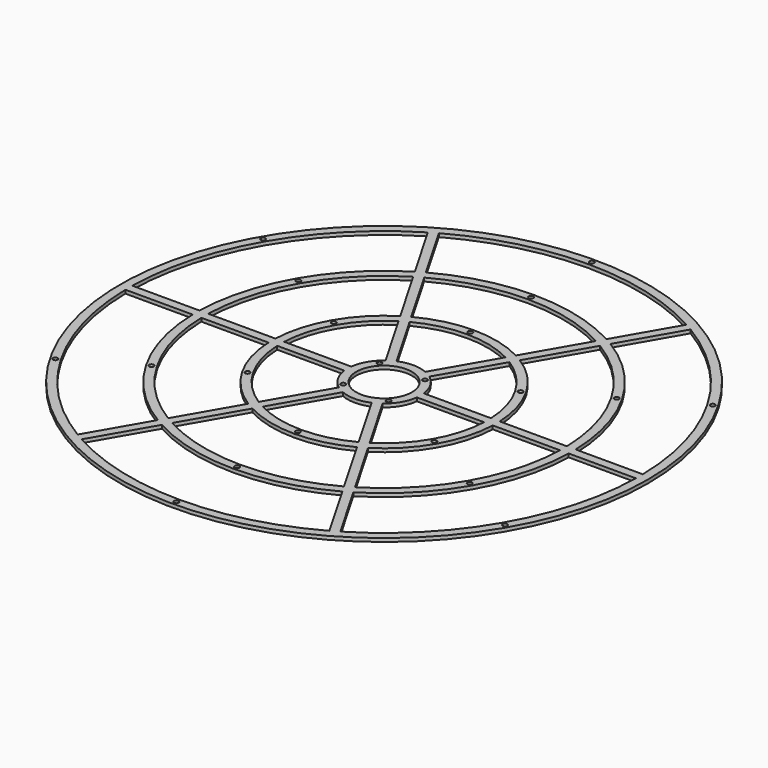
from build123d import *

# Parameters (mm, degrees)
F0_R            = 241.3
F0_R_2          = 25.4
F1_DEPTH        = 3.175
F2_R            = 2.15265
F3_DEPTH        = 3.175
F3_COPIES_COUNT = 6
F4_R            = 2.15265
F5_DEPTH        = 3.175


# Not quite as in the source:
# - a pattern or mirror of a feature is missing from the dataset's text; its kind, count and spacing are read off the source's solid


with BuildPart() as f1:
    # F0 (on Top) → F1 (new body)
    with BuildSketch(Plane.XY):
        Circle(F0_R)
        Circle(F0_R_2, mode=Mode.SUBTRACT)
    extrude(amount=F1_DEPTH)

    # F2 (on face) → F3 (cut, through all)
    with BuildSketch(Plane.XY.offset(3.175)):
        with BuildLine():
            ThreePointArc((13.1131726267, -30.6501812378), (0, -33.3375), (-13.1131726267, -30.6501812378))
            Line((-13.1131726267, -30.6501812378), (-43.8387272582, -83.8684029504))
            ThreePointArc((-43.8387272582, -83.8684029504), (0, -94.6347875841), (43.8387272582, -83.8684029504))
            Line((43.8387272582, -83.8684029504), (13.1131726267, -30.6501812378))
        make_face()
        with BuildLine():
            Line((-82.5017818898, -150.8347779481), (-113.2273365214, -204.0529996607))
            ThreePointArc((-113.2273365214, -204.0529996607), (0, -233.3625), (113.2273365214, -204.0529996607))
            Line((113.2273365214, -204.0529996607), (82.5017818898, -150.8347779481))
            ThreePointArc((82.5017818898, -150.8347779481), (0, -171.923454635), (-82.5017818898, -150.8347779481))
        make_face()
        with BuildLine():
            ThreePointArc((47.8074772582, -90.742479593), (0, -102.5658446291), (-47.8074772582, -90.742479593))
            Line((-47.8074772582, -90.742479593), (-78.5330318898, -143.9607013056))
            ThreePointArc((-78.5330318898, -143.9607013056), (0, -163.9881721899), (78.5330318898, -143.9607013056))
            Line((78.5330318898, -143.9607013056), (47.8074772582, -90.742479593))
        make_face()
        with Locations((0, -98.6003161066)):
            Circle(F2_R)
        with Locations((0, -167.9558134125)):
            Circle(F2_R)
        with Locations((0, -237.33125)):
            Circle(F2_R)
    f3 = extrude(amount=-F3_DEPTH, mode=Mode.SUBTRACT)

    # F3_copies: F3 ×6 about axis
    f3_copies_axis = Axis((0, 0, 0), (0, 0, 1))
    for i in range(1, F3_COPIES_COUNT):
        add(f3.rotate(f3_copies_axis, i * 360 / F3_COPIES_COUNT), mode=Mode.SUBTRACT)

    # F4 (on face) → F5 (cut, through all)
    with BuildSketch(Plane.XY.offset(3.175)):
        with Locations((-20.76684228, 20.76684228)):
            Circle(F4_R)
        with Locations((20.76684228, 20.76684228)):
            Circle(F4_R)
        with Locations((20.76684228, -20.76684228)):
            Circle(F4_R)
        with Locations((-20.76684228, -20.76684228)):
            Circle(F4_R)
    extrude(amount=-F5_DEPTH, mode=Mode.SUBTRACT)


solid = f1.part
